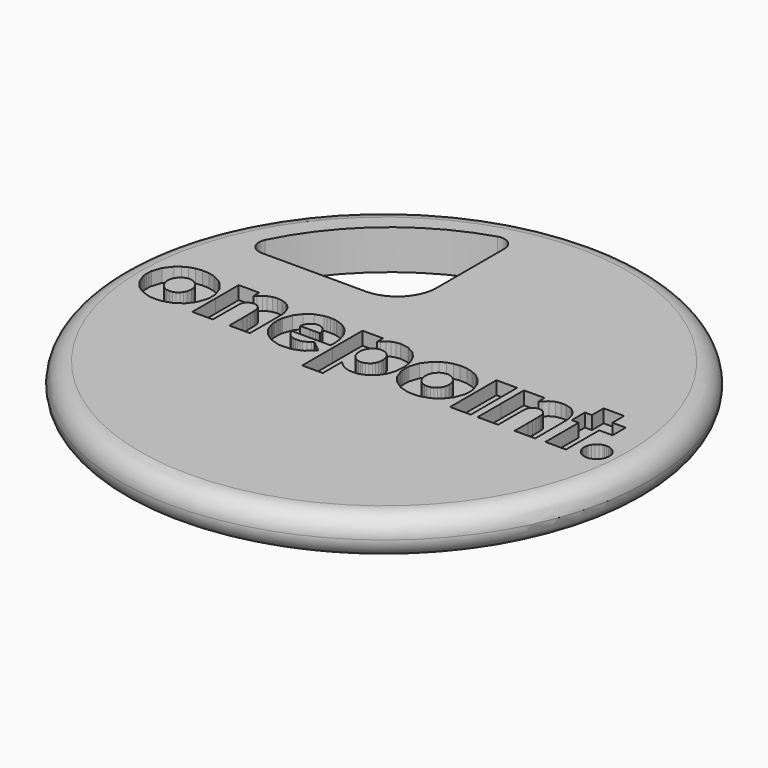
from build123d import *

# Parameters (mm, degrees)
F0_R     = 20
F1_DEPTH = 3
F3_DEPTH = 1
F5_DEPTH = 3.001
F6_R     = 3
F7_R     = 1
F8_R     = 1.49999


# Not quite as in the source:
# - a fillet or chamfer is up to 0.001 mm smaller than in the source, because OpenCascade refuses the exact size


with BuildPart() as f1:
    # F0 (on Top) → F1 (new body)
    with BuildSketch(Plane.XY):
        Circle(F0_R)
    extrude(amount=F1_DEPTH)

    # F2 (on face) → F3 (cut)
    with BuildSketch(Plane.XY.offset(3)):
        Polygon((-16.6981611057, -1.9646729061), (-15.9984856655, -2.1771155881), (-15.9984856655, -2.1773510687), (-15.5641104362, -2.1990545239), (-15.121438443, -2.1669506787), (-14.4266531484, -1.9433226717), (-13.8498357484, -1.5411219317), (-13.4239809895, -0.9900974987), (-13.1816676026, -0.3199984127), (-13.1567576876, -0.1315747444), (-13.145470321, 0.0877753664), (-13.1497325185, 0.3070862305), (-13.1710238828, 0.495313665), (-13.4005585264, 1.1555618157), (-13.8313112803, 1.7230698855), (-14.2245873082, 2.0281741549), (-14.6710937093, 2.2443060318), (-15.16210593, 2.3673838539), (-15.6886757102, 2.3937576729), (-16.1462536208, 2.333945619), (-16.5708328601, 2.2014878227), (-16.9568678619, 1.9977579201), (-17.2981890363, 1.7230698855), (-17.7472543258, 1.1324062305), (-17.9793439331, 0.4333037929), (-17.9965928817, 0.2395818127), (-17.9999995, 0.0194467668), (-17.9882882685, -0.1948012659), (-17.9589042234, -0.3714901546), (-17.7063749063, -1.0366833963), (-17.2766857395, -1.5760515432), align=None)
        Polygon((-15.1312305083, -0.7728667127), (-15.338198268, -0.8563838062), (-15.3384102005, -0.8563838062), (-15.5692242883, -0.8795393914), (-15.7923695603, -0.8563838062), (-16.0189253752, -0.7596798032), (-16.211623015, -0.6023395644), (-16.3596107522, -0.3964118437), (-16.4526569577, -0.1547695763), (-16.4762913533, -0.0406400143), (-16.4839562444, 0.1007660421), (-16.4762913533, 0.2457435532), (-16.4526569577, 0.3714116611), (-16.3889908726, 0.5551649656), (-16.2825262017, 0.7261630748), (-16.1451900337, 0.8719647678), (-15.9882658106, 0.9801680699), (-15.7834291496, 1.0512439422), (-15.5860454473, 1.0833870342), (-15.5100284085, 1.0757731638), (-15.4105928313, 1.0523428514), (-15.1716860628, 0.9665494461), (-14.9696202226, 0.8215326882), (-14.8099251786, 0.6245532275), (-14.6985625128, 0.381812051), (-14.6627930208, 0.0658364306), (-14.7190022225, -0.2580277874), (-14.8216324855, -0.4747876124), (-14.9589725781, -0.6461781892), align=None, mode=Mode.SUBTRACT)
        Polygon((-12.8307662955, 2.269855669), (-12.8307662955, 0.0721944049), (-12.8311901604, 0.0721944049), (-12.8311901604, -2.1256238462), (-11.2732117476, -2.1256238462), (-11.2732117476, -0.8254573637), (-11.2699935138, -0.4019848828), (-11.267246241, -0.0810641714), (-11.2644597214, 0.1531604594), (-11.2610452538, 0.3160344905), (-11.2566103705, 0.4233351172), (-11.2508410976, 0.4906040544), (-11.2429524999, 0.5333830168), (-11.23255211, 0.5674491997), (-11.1237208598, 0.7539890238), (-10.9734057901, 0.889822041), (-10.7900841999, 0.968001576), (-10.5824688687, 0.9801680699), (-10.4061724476, 0.941627757), (-10.2628433002, 0.856423053), (-10.1502051148, 0.7248286852), (-10.0665310343, 0.5468054069), (-10.0563268781, 0.5095994836), (-10.0484382805, 0.4642302354), (-10.0427082543, 0.3954306748), (-10.0379986438, 0.2877375805), (-10.0345841761, 0.1252167702), (-10.0316014228, -0.1074772372), (-10.0284224357, -0.4260038965), (-10.0248117343, -0.8461404033), (-10.0248117343, -2.1256238462), (-8.4667940747, -2.1256238462), (-8.4667940747, -0.5365227572), (-8.4702477891, -0.0676810281), (-8.472995062, 0.3028083342), (-8.4757423348, 0.587700525), (-8.4791568024, 0.7995545057), (-8.4836309324, 0.9518319131), (-8.4893609586, 1.0568169814), (-8.4972495562, 1.1272649057), (-8.5074537124, 1.1762448553), (-8.6167166769, 1.5352349185), (-8.7772751495, 1.8262888498), (-8.993799494, 2.055646883), (-9.2710385676, 2.2285288365), (-9.6029876171, 2.3388514634), (-9.9598583556, 2.3744090229), (-10.3131183927, 2.3345735671), (-10.6331364288, 2.2183246803), (-10.8782324105, 2.0777428058), (-11.1077474307, 1.8674194485), (-11.2727800333, 1.7024260926), (-11.2727800333, 2.269855669), align=None)
        Polygon((-6.9818538721, -1.9784877637), (-6.2479003165, -2.1977986277), (-6.2466444203, -2.1977986277), (-6.1817302884, -2.2050592773), (-6.0739587006, -2.2105538229), (-5.9391460989, -2.2120844464), (-5.7926772112, -2.2080420307), (-5.5942063738, -2.2059227059), (-5.4575099279, -2.1988975369), (-5.3517006778, -2.1862993287), (-5.2458914277, -2.1669506787), (-4.5610748087, -1.8920664103), (-4.0076955705, -1.4240488631), (-3.9250811523, -1.3309948082), (-4.3583653218, -0.9698461734), (-4.7918849719, -0.6087367854), (-4.9156299888, -0.7119949965), (-5.1479315285, -0.8834248201), (-5.3800368346, -1.000929603), (-5.5267412028, -1.0333081754), (-5.7013107668, -1.0512046955), (-5.8778034217, -1.0516364098), (-6.0300808291, -1.031777552), (-6.2208593026, -0.9647440954), (-6.3873832819, -0.8601907414), (-6.5249039096, -0.7226701137), (-6.6283976012, -0.55716655), (-6.6712158103, -0.4641124952), (-6.6905644603, -0.4024165971), (-6.701475058, -0.3610897646), (-3.7813202907, -0.3610897646), (-3.7609119783, -0.2269443578), (-3.7609119783, -0.0570451576), (-3.7728429917, 0.1716849275), (-3.7945856937, 0.4101482077), (-3.8230788374, 0.6087760322), (-4.0411338053, 1.2473599744), (-4.3905476605, 1.754153315), (-4.8704962211, 2.1242109631), (-5.4739150713, 2.3318262943), (-5.6860045325, 2.3609866329), (-5.9472701771, 2.3718579839), (-6.2067697178, 2.3652252824), (-6.4129329191, 2.3422266842), (-7.0295386788, 2.1280178983), (-7.5376271623, 1.7437136784), (-7.928524837, 1.2188668306), (-8.1565877273, 0.5777318494), (-8.1757793902, 0.478516054), (-8.1882991049, 0.3780051158), (-8.195324274, 0.2485300728), (-8.1974828455, 0.0617940149), (-8.1955597545, -0.1202716791), (-8.1887308192, -0.2501784365), (-8.1761718578, -0.3529656865), (-8.1565877273, -0.4541438195), (-7.9441057985, -1.0601137087), (-7.5687105919, -1.5581942699), align=None)
        Polygon((-5.236903921, 0.5410753807), (-5.2262680505, 0.4746306254), (-5.226503531, 0.4746306254), (-5.230977661, 0.4678409368), (-5.24840322, 0.4627388587), (-5.2852559225, 0.4590889106), (-5.3478937426, 0.4567733521), (-5.4421644469, 0.4552819754), (-5.5748577238, 0.4544185468), (-5.751782093, 0.4541830663), (-5.9796487496, 0.4539868325), (-6.7329509551, 0.4539868325), (-6.7019067723, 0.5777318494), (-6.6053990031, 0.8215326882), (-6.4710573625, 1.0099956033), (-6.3000592532, 1.1423749061), (-6.0931503635, 1.217532441), (-5.8637530836, 1.2188668306), (-5.6506432067, 1.1492038414), (-5.4707360842, 1.0159218632), (-5.3397696645, 0.8253396234), (-5.3005621567, 0.73589627), (-5.2639841816, 0.6345611499), align=None, mode=Mode.SUBTRACT)
        Polygon((-3.4619694494, 2.2802560589), (-3.4619694494, -0.5676454335), (-3.4621656832, -0.5676454335), (-3.4621656832, -3.4257118353), (-1.9039910367, -3.4257118353), (-1.9039910367, -1.6096860118), (-1.7802460198, -1.7231876258), (-1.60308617, -1.8809988255), (-1.4229828137, -2.0029777385), (-1.2332247558, -2.0960317934), (-1.0269045674, -2.1669506787), (-0.931534954, -2.1907734587), (-0.8427195486, -2.2029007058), (-0.7326716491, -2.2073748358), (-0.5729766051, -2.2081990177), (-0.4194825483, -2.2073748358), (-0.3112792462, -2.2029007058), (-0.2205799966, -2.1907734587), (-0.119009396, -2.1669506787), (0.3864888018, -1.9437936327), (0.8069785293, -1.582644998), (1.1229933964, -1.1033636322), (1.3153024934, -0.526318601), (1.3706011705, 0.1973915517), (1.263732258, 0.8975144049), (0.9737379891, 1.5258549442), (0.5310738453, 1.99921005), (-0.0276429515, 2.2907349424), (-0.6657951794, 2.3730746333), (-0.9775321503, 2.3319832813), (-1.2554384188, 2.2364566809), (-1.5117982191, 2.0828841306), (-1.7594059931, 1.8674194485), (-1.9039910367, 1.7128264826), (-1.9039910367, 2.2802560589), align=None)
        Polygon((-0.7237233891, -0.8472000657), (-0.9030025635, -0.8976713919), (-1.066936257, -0.9130168729), (-1.2230598464, -0.8976713919), (-1.4512797237, -0.8082280385), (-1.6473957558, -0.6551264492), (-1.7990059684, -0.4477858453), (-1.8935514, -0.196057162), (-1.9165107513, -0.071056249), (-1.9242031152, 0.0826732883), (-1.9165107513, 0.2363635789), (-1.8935514, 0.3611682581), (-1.7893905136, 0.6202753312), (-1.6254960668, 0.8319330782), (-1.4148587355, 0.9835432908), (-1.1713326239, 1.0627432413), (-0.8487243021, 1.0461811109), (-0.5627332022, 0.9145867431), (-0.3385164938, 0.6841690475), (-0.2014275804, 0.3714116611), (-0.1664979689, 0.1627366675), (-0.1692844885, -0.0528065082), (-0.208845217, -0.2626981511), (-0.2840027518, -0.4541438195), (-0.399859171, -0.6146630454), (-0.5510376693, -0.7492794132), align=None, mode=Mode.SUBTRACT)
        Polygon((6.6910481954, 2.2802560589), (6.6910481954, 0.0824378078), (6.6910481954, -2.1151449628), (8.2594662448, -2.1151449628), (8.2594662448, 2.2802560589), align=None)
        Polygon((2.8340733984, -1.9646729061), (3.5337645374, -2.1771155881), (3.968147616, -2.1990545239), (4.4106155261, -2.1669506787), (5.1054008207, -1.9433226717), (5.6822103714, -1.5411219317), (6.1082338913, -0.9900974987), (6.3505826002, -0.3199984127), (6.3755042893, -0.1315747444), (6.3868073546, 0.0877753664), (6.3825294584, 0.3070862305), (6.3612184707, 0.495313665), (6.1314679699, 1.1555618157), (5.7007348395, 1.7230698855), (5.3074431128, 2.0281741549), (4.8611290208, 2.2443060318), (4.3701521222, 2.3673838539), (3.8435391705, 2.3937576729), (3.3860005068, 2.333945619), (2.9614291167, 2.2014878227), (2.5753980396, 1.9977579201), (2.2340297691, 1.7230698855), (1.7850076511, 1.1324062305), (1.5529023451, 0.4333037929), (1.5356730198, 0.2395818127), (1.5320230717, 0.0194467668), (1.543954085, -0.1948012659), (1.5733499042, -0.3714901546), (1.8258635225, -1.0366833963), (2.2555762374, -1.5760515432), align=None)
        Polygon((4.4010000712, -0.7728667127), (4.1940519348, -0.8563838062), (4.1938164543, -0.8563838062), (3.9630455379, -0.8795393914), (3.7398884919, -0.8563838062), (3.5133169783, -0.7596798032), (3.3206546605, -0.6023395644), (3.1724196689, -0.3964118437), (3.0796010945, -0.1547695763), (3.0559353015, -0.0406400143), (3.0483214312, 0.1007660421), (3.0559353015, 0.2457435532), (3.0796010945, 0.3714116611), (3.1432593303, 0.5551649656), (3.2497357752, 0.7261630748), (3.3870209224, 0.8719647678), (3.543733213, 0.9801680699), (3.7487975052, 1.0512439422), (3.9461694335, 1.0833870342), (4.0219941632, 1.0757731638), (4.1216416728, 1.0523428514), (4.3603404336, 0.9665494461), (4.5626182062, 0.8215326882), (4.7221170164, 0.6245532275), (4.8334993056, 0.381812051), (4.8694493328, 0.0658364306), (4.8132087336, -0.2580277874), (4.7106177174, -0.4747876124), (4.5732540767, -0.6461781892), align=None, mode=Mode.SUBTRACT)
        Polygon((8.7754040793, 2.2802560589), (8.7754040793, 0.0824378078), (8.7745014039, 0.0824378078), (8.7745014039, -2.1151449628), (10.3325190634, -2.1151449628), (10.3325190634, -0.887427989), (10.3325190634, -0.4522207285), (10.3338142063, -0.1189765362), (10.3367969597, 0.1286704846), (10.3427624664, 0.3070862305), (10.352574155, 0.4320478967), (10.3672131944, 0.5201961073), (10.3876607535, 0.5873080575), (10.4149372479, 0.6499066309), (10.536091979, 0.8176865063), (10.7041073349, 0.9388412374), (10.9323272122, 0.9961414989), (11.1540321283, 0.9699246669), (11.3466944461, 0.8664702221), (11.4881005025, 0.6911942166), (11.5187522177, 0.6328735394), (11.5419470496, 0.569804005), (11.5585876735, 0.4848740283), (11.5696552583, 0.3611682581), (11.576248713, 0.1812218888), (11.5798594145, -0.0717234438), (11.5811545574, -0.4154072728), (11.5813507911, -0.8667841962), (11.5813507911, -2.1151449628), (13.1395254377, -2.1151449628), (13.1395254377, -0.5882892263), (13.1378378272, 0.0340858063), (13.1331282167, 0.5429984717), (13.1267702425, 0.8992020154), (13.1191171253, 1.0627432413), (12.985364186, 1.5618834648), (12.7309274767, 1.9526241525), (12.3662073873, 2.2234267584), (11.9017612947, 2.3626742433), (11.508312581, 2.3782159581), (11.1456725696, 2.2996832024), (10.8103482993, 2.1263302878), (10.4983758479, 1.8572152923), (10.333382492, 1.692143443), (10.333382492, 2.2802560589), align=None)
        Polygon((13.8929061367, 1.0627432413), (13.8929061367, -0.5159182111), (13.8929061367, -2.0842970138), (15.4508845495, -2.0842970138), (15.4508845495, 1.0627432413), (16.4623126593, 1.0627432413), (16.4623126593, 2.3111825014), (15.4508845495, 2.3111825014), (15.4508845495, 3.4257118353), (13.8929061367, 3.4257118353), (13.8929061367, 2.3111825014), (13.3667248994, 2.3111825014), (13.3667248994, 1.0627432413), align=None)
        Polygon((16.5610574936, -1.9886919198), (16.8027782545, -2.0946974037), (16.803170722, -2.0946974037), (16.9107068293, -2.1120052224), (17.0465398466, -2.1177352486), (17.1845706821, -2.1120052224), (17.2984255168, -2.0946974037), (17.5777839153, -1.9669884646), (17.8000775327, -1.7553307177), (17.9468211477, -1.4836646831), (18.0000005, -1.1764018423), (17.9529828881, -0.8746727938), (17.8182095332, -0.6125437206), (17.6038045135, -0.4028090646), (17.3190693097, -0.2580277874), (17.2003086306, -0.2345974749), (17.0505822623, -0.2269443578), (16.9010913744, -0.2345974749), (16.7825661759, -0.2580277874), (16.5678864289, -0.3543000761), (16.3902948648, -0.4875428076), (16.2514790942, -0.6555581635), (16.153362208, -0.8563838062), (16.1216115836, -0.9672951344), (16.1050102065, -1.1014405412), (16.1017919726, -1.2393928832), (16.1113681807, -1.362038991), (16.2018711966, -1.6068994922), (16.3564641625, -1.821147525), align=None)
    extrude(amount=-F3_DEPTH, mode=Mode.SUBTRACT)

    # F4 (on face) → F5 (cut, through all)
    with BuildSketch(Plane.XY.offset(3)):
        with BuildLine():
            Line((-3.4619694494, 6.3287522644), (-3.4619694494, 17.0396789908))
            ThreePointArc((-3.4619694494, 17.0396789908), (-10.995184255, 13.2278056663), (-15.8616784457, 6.3287522644))
            Line((-15.8616784457, 6.3287522644), (-3.4619694494, 6.3287522644))
        make_face()
    extrude(amount=-F5_DEPTH, mode=Mode.SUBTRACT)

    # F6
    f6_edges = [f1.edges().sort_by_distance(p)[0] for p in [
        (-3.461969, 6.328752, 1.5),
    ]]
    fillet(f6_edges, radius=F6_R)

    # F7
    f7_edges = [f1.edges().sort_by_distance(p)[0] for p in [
        (-3.461969, 17.039679, 1.5),
        (-15.861678, 6.328752, 1.5),
    ]]
    fillet(f7_edges, radius=F7_R)

    # F8 (radius 1.5 in the source; OpenCascade refuses exactly that, so slightly less here)
    f8_edges = [f1.edges().sort_by_distance(p)[0] for p in [
        (-20, 0, 3),
        (-20, 0, 0),
    ]]
    fillet(f8_edges, radius=F8_R)


solid = f1.part
